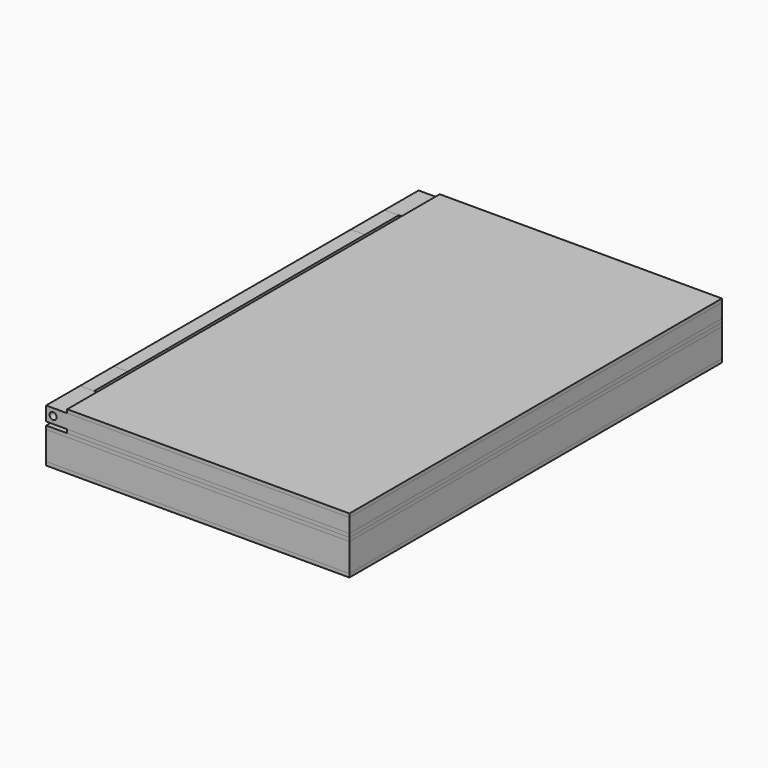
from build123d import *

# Parameters (mm, degrees)
F0_W      = 215
F0_H      = 330
F1_DEPTH  = 2.5
F2_W      = 215
F2_H      = 330
F2_W_2    = 195
F2_H_2    = 310
F3_DEPTH  = 20
F4_R      = 2.5
F5_DEPTH  = 30
F8_W      = 215
F8_H      = 330
F9_DEPTH  = 2.5
F11_W     = 200
F11_H     = 330
F11_W_2   = 170
F11_H_2   = 300
F12_DEPTH = 2.5
F13_W     = 180
F13_H     = 310
F14_DEPTH = 10
F15_W     = 200
F15_H     = 330
F16_DEPTH = 2.5
F17_R     = 2.5
F18_DEPTH = 999
F20_DEPTH = 210


with BuildPart() as f1:
    # F0 (on Top) → F1 (new body)
    with BuildSketch(Plane.XY):
        with Locations((107.5, 165)):
            Rectangle(F0_W, F0_H)
    extrude(amount=F1_DEPTH)


with BuildPart() as f3:
    # F2 (on face) → F3 (new body)
    with BuildSketch(Plane.XY.offset(2.5)):
        with Locations((107.5, 165)):
            Rectangle(F2_W, F2_H)
        with Locations((107.5, 165)):
            Rectangle(F2_W_2, F2_H_2, mode=Mode.SUBTRACT)
    extrude(amount=F3_DEPTH)


with BuildPart() as f5:
    # F4 (on Front) → F5 (new body)
    with BuildSketch(Plane.XZ):
        Polygon((0, 2.5), (0, 0), (0, -2.5), (10, -2.5), (10, 37.5), (0, 37.5), (0, 22.5), (5, 22.5), (5, 2.5), align=None)
        with Locations((5, 32.5)):
            Circle(F4_R, mode=Mode.SUBTRACT)
    extrude(amount=-F5_DEPTH)


with BuildPart() as f5_1:
    # F6: moved
    add(f5.part.moved(Location((0, 30, 0))))


with BuildPart() as f7_1:
    # F7: copy of F5
    add(f5_1.part.moved(Location((0, 240, 0))))


with BuildPart() as f9:
    # F8 (on face) → F9 (new body)
    with BuildSketch(Plane.XY.offset(22.5)):
        with Locations((107.5, 165)):
            Rectangle(F8_W, F8_H)
    extrude(amount=F9_DEPTH)

    # F10: cut F7_1, F5
    add(f7_1.part, mode=Mode.SUBTRACT)
    add(f5_1.part, mode=Mode.SUBTRACT)


with BuildPart() as f3_1:
    add(f3.part)

    # F10: cut F7_1, F5
    add(f7_1.part, mode=Mode.SUBTRACT)
    add(f5_1.part, mode=Mode.SUBTRACT)


with BuildPart() as f1_1:
    add(f1.part)

    # F10: cut F7_1, F5
    add(f7_1.part, mode=Mode.SUBTRACT)
    add(f5_1.part, mode=Mode.SUBTRACT)


with BuildPart() as f12:
    # F11 (on face) → F12 (new body)
    with BuildSketch(Plane.XY.offset(25)):
        with Locations((115, 165)):
            Rectangle(F11_W, F11_H)
        with Locations((115, 165)):
            Rectangle(F11_W_2, F11_H_2, mode=Mode.SUBTRACT)
    extrude(amount=F12_DEPTH)


with BuildPart() as f14:
    # F13 (on face) → F14 (new body)
    with BuildSketch(Plane.XY.offset(27.5)):
        Polygon((0, 0), (215, 0), (215, 330), (0, 330), (0, 300), (15, 300), (15, 30), (0, 30), align=None)
        with Locations((115, 165)):
            Rectangle(F13_W, F13_H, mode=Mode.SUBTRACT)
    extrude(amount=F14_DEPTH)

    # F17 (on face) → F18 (cut)
    with BuildSketch(Plane.XZ):
        with Locations((5, 32.5)):
            Circle(F17_R)
    extrude(amount=-F18_DEPTH, mode=Mode.SUBTRACT)


with BuildPart() as f16:
    # F15 (on face) → F16 (new body)
    with BuildSketch(Plane.XY.offset(37.5)):
        with Locations((115, 165)):
            Rectangle(F15_W, F15_H)
    extrude(amount=F16_DEPTH)


with BuildPart() as f20:
    # F19 (on face) → F20 (new body, through all)
    with BuildSketch(Plane.XZ.offset(-270)):
        Polygon((10, 37.5), (0, 37.5), (0, 25), (1, 25), (1, 36.5), (9, 36.5), (9, 25), (10, 25), align=None)
    extrude(amount=F20_DEPTH)


solid = Compound([f5_1.part, f7_1.part, f9.part, f3_1.part, f1_1.part, f12.part, f14.part, f16.part, f20.part])
